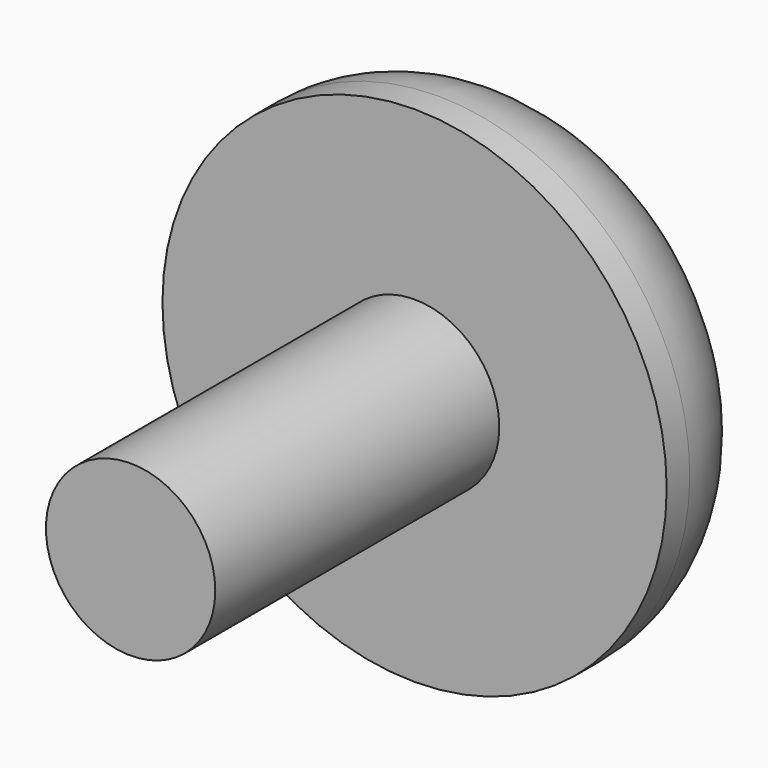
from build123d import *

# Parameters (mm, degrees)
F0_R     = 3.7317681235
F1_DEPTH = 15.6464
F0_R_2   = 11.1125
F2_DEPTH = 6.35
F3_R     = 5.08
F4_DEPTH = 6.35


with BuildPart() as f1:
    # F0 (on Front) → F1 (new body)
    with BuildSketch(Plane.XZ):
        Circle(F0_R)
    extrude(amount=F1_DEPTH)

    # F4 (add, through all): a face of the model
    f4_faces = [f1.faces().sort_by_distance(p)[0] for p in [
        (0, 0, 0),
    ]]
    extrude(f4_faces, amount=F4_DEPTH)


with BuildPart() as f2:
    # F0 (on Front) → F2 (new body)
    with BuildSketch(Plane.XZ):
        Circle(F0_R_2)
        Circle(F0_R, mode=Mode.SUBTRACT)
    extrude(amount=-F2_DEPTH)

    # F3
    f3_edges = [f2.edges().sort_by_distance(p)[0] for p in [
        (-11.1125, 6.35, 0),
    ]]
    fillet(f3_edges, radius=F3_R)


solid = Compound([f1.part, f2.part])
